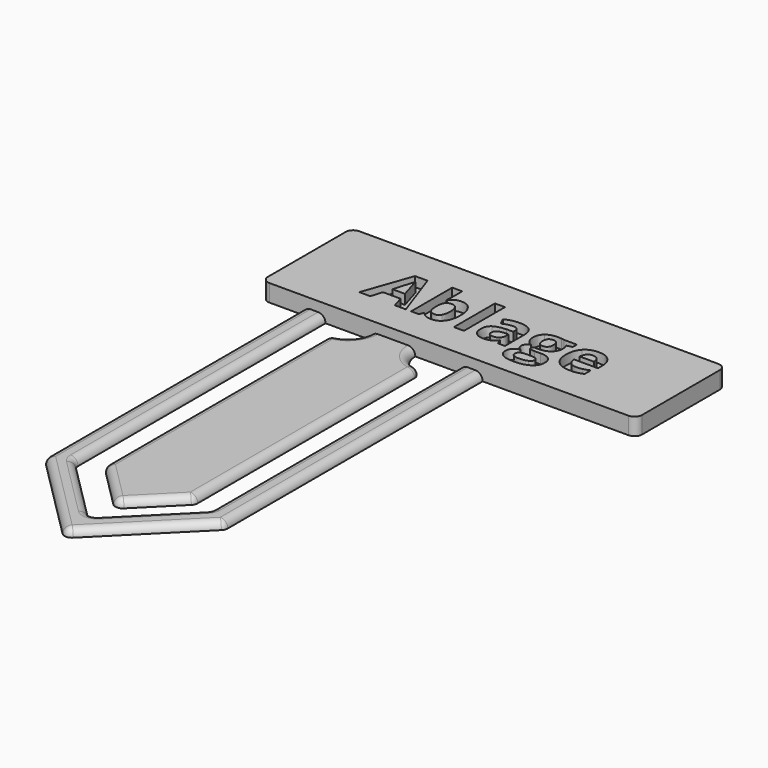
from build123d import *

# Parameters (mm, degrees)
F0_TEXT_SIZE = 9.0277777778
F1_DEPTH     = 1
F0_W         = 1.3442925347
F0_H         = 6.8597005208
F2_DEPTH     = 2.3
F3_R         = 0.99999


# Not quite as in the source:
# - a fillet or chamfer is up to 0.001 mm smaller than in the source, because OpenCascade refuses the exact size
# - Text() gives the source's letters only with a copy of the font that has no kerning and outlines rounded to 1/6400 em; it was checked with that copy


with BuildPart() as f1:
    # F0 (on Top) → F1 (new body)
    with BuildSketch(Plane.XY):
        Polygon((-11.1783012444, 18.0121831276), (-14.1783012444, 18.0121831276), (-14.1783012444, -24.9878168724), (-2.1783012444, -36.9878168724), (9.8216987556, -24.9878168724), (9.8216987556, 18.0121831276), (6.8216987556, 18.0121831276), (6.8216987556, -23.7451761852), (-2.1783012444, -32.7451761852), (-11.1783012444, -23.7451761852), align=None)
        with BuildLine():
            Line((0.8216987556, 18.0121831276), (-5.1783012444, 18.0121831276))
            ThreePointArc((-5.1783012444, 18.0121831276), (-6.0569809009, 15.8908627841), (-8.1783012444, 15.0121831276))
            Line((-8.1783012444, 15.0121831276), (-8.1783012444, -22.5025354981))
            Line((-8.1783012444, -22.5025354981), (-2.1783012444, -28.5025354981))
            Line((-2.1783012444, -28.5025354981), (3.8216987556, -22.5025354981))
            Line((3.8216987556, -22.5025354981), (3.8216987556, 15.0121831276))
            ThreePointArc((3.8216987556, 15.0121831276), (1.700378412, 15.8908627841), (0.8216987556, 18.0121831276))
        make_face()
        with Locations((-10.0730566365, 22.2621831276)):
            Text('Ablage', F0_TEXT_SIZE, font='Open Sans', font_style=FontStyle.BOLD, text_align=(TextAlign.LEFT, TextAlign.BOTTOM))
    extrude(amount=F1_DEPTH)

    # F0 (on Top) → F2 (join)
    with BuildSketch(Plane.XY):
        Polygon((-19.6821061156, 18.0121831276), (-14.1783012444, 18.0121831276), (-11.1783012444, 18.0121831276), (-5.1783012444, 18.0121831276), (0.8216987556, 18.0121831276), (6.8216987556, 18.0121831276), (9.8216987556, 18.0121831276), (30.3178938844, 18.0121831276), (30.3178938844, 33.0121831276), (-19.6821061156, 33.0121831276), align=None)
        Polygon((-3.8438899698, 22.2621831276), (-5.3165462198, 22.2621831276), (-5.7834516017, 23.7969053499), (-8.1334950045, 23.7969053499), (-8.6004003865, 22.2621831276), (-10.0730566365, 22.2621831276), (-7.7977745184, 28.7339713221), (-6.1276356295, 28.7339713221), align=None, mode=Mode.SUBTRACT)
        with BuildLine():
            add(Edge.make_bspline(
                [(-1.7943022962, 26.5517881624), (-1.3217545531, 27.2824739263), (-0.3964073309, 27.2824739263)],
                knots=[0, 0, 0, 1, 1, 1], degree=2))
            add(Edge.make_bspline(
                [(-0.3964073309, 27.2824739263), (0.476748051, 27.2824739263), (0.9704546483, 26.6018641172)],
                knots=[0, 0, 0, 1, 1, 1], degree=2))
            add(Edge.make_bspline(
                [(0.9704546483, 26.6018641172), (1.4641612455, 25.9212543082), (1.4641612455, 24.7349478846)],
                knots=[0, 0, 0, 1, 1, 1], degree=2))
            add(Edge.make_bspline(
                [(1.4641612455, 24.7349478846), (1.4641612455, 23.5147872943), (0.9549381552, 22.8440516172)],
                knots=[0, 0, 0, 1, 1, 1], degree=2))
            add(Edge.make_bspline(
                [(0.9549381552, 22.8440516172), (0.4457150649, 22.1733159401), (-0.4316720878, 22.1733159401)],
                knots=[0, 0, 0, 1, 1, 1], degree=2))
            add(Edge.make_bspline(
                [(-0.4316720878, 22.1733159401), (-1.300595699, 22.1733159401), (-1.7943022962, 22.8038497943)],
                knots=[0, 0, 0, 1, 1, 1], degree=2))
            Line((-1.7943022962, 22.8038497943), (-1.8859906642, 22.8038497943))
            Line((-1.8859906642, 22.8038497943), (-2.1116851087, 22.2621831276))
            Line((-2.1116851087, 22.2621831276), (-3.1385948309, 22.2621831276))
            Line((-3.1385948309, 22.2621831276), (-3.1385948309, 29.1218836485))
            Line((-3.1385948309, 29.1218836485), (-1.7943022962, 29.1218836485))
            Line((-1.7943022962, 29.1218836485), (-1.7943022962, 27.525095454))
            add(Edge.make_bspline(
                [(-1.7943022962, 27.525095454), (-1.7943022962, 27.2218185443), (-1.8464941365, 26.5517881624)],
                knots=[0, 0, 0, 1, 1, 1], degree=2))
            Line((-1.8464941365, 26.5517881624), (-1.7943022962, 26.5517881624))
        make_face(mode=Mode.SUBTRACT)
        with Locations((3.2464420615, 25.6920333881)):
            Rectangle(F0_W, F0_H, mode=Mode.SUBTRACT)
        with BuildLine():
            Line((13.3526161066, 27.1907855582), (15.0721256552, 27.1907855582))
            Line((15.0721256552, 27.1907855582), (15.0721256552, 26.5066492735))
            Line((15.0721256552, 26.5066492735), (14.3005327733, 26.3091666346))
            add(Edge.make_bspline(
                [(14.3005327733, 26.3091666346), (14.5121213149, 25.9776779193), (14.5121213149, 25.5686067388)],
                knots=[0, 0, 0, 1, 1, 1], degree=2))
            add(Edge.make_bspline(
                [(14.5121213149, 25.5686067388), (14.5121213149, 24.7744444124), (13.9584646309, 24.3315190651)],
                knots=[0, 0, 0, 1, 1, 1], degree=2))
            add(Edge.make_bspline(
                [(13.9584646309, 24.3315190651), (13.4048079469, 23.8885937179), (12.4230371135, 23.8885937179)],
                knots=[0, 0, 0, 1, 1, 1], degree=2))
            Line((12.4230371135, 23.8885937179), (12.1804155858, 23.9026996207))
            Line((12.1804155858, 23.9026996207), (11.9815223566, 23.9238584749))
            add(Edge.make_bspline(
                [(11.9815223566, 23.9238584749), (11.7741655858, 23.7658723638), (11.7741655858, 23.5712109054)],
                knots=[0, 0, 0, 1, 1, 1], degree=2))
            add(Edge.make_bspline(
                [(11.7741655858, 23.5712109054), (11.7741655858, 23.2806293082), (12.5147254816, 23.2806293082)],
                knots=[0, 0, 0, 1, 1, 1], degree=2))
            Line((12.5147254816, 23.2806293082), (13.3526161066, 23.2806293082))
            add(Edge.make_bspline(
                [(13.3526161066, 23.2806293082), (14.1637055163, 23.2806293082), (14.5889984851, 22.9322135096)],
                knots=[0, 0, 0, 1, 1, 1], degree=2))
            add(Edge.make_bspline(
                [(14.5889984851, 22.9322135096), (15.0142914538, 22.583797711), (15.0142914538, 21.9095355582)],
                knots=[0, 0, 0, 1, 1, 1], degree=2))
            add(Edge.make_bspline(
                [(15.0142914538, 21.9095355582), (15.0142914538, 21.0448437179), (14.2934798219, 20.5687694992)],
                knots=[0, 0, 0, 1, 1, 1], degree=2))
            add(Edge.make_bspline(
                [(14.2934798219, 20.5687694992), (13.5726681899, 20.0926952804), (12.2241438844, 20.0926952804)],
                knots=[0, 0, 0, 1, 1, 1], degree=2))
            add(Edge.make_bspline(
                [(12.2241438844, 20.0926952804), (11.1930023913, 20.0926952804), (10.6485145441, 20.4523958013)],
                knots=[0, 0, 0, 1, 1, 1], degree=2))
            add(Edge.make_bspline(
                [(10.6485145441, 20.4523958013), (10.1040266969, 20.8120963221), (10.1040266969, 21.4595572596)],
                knots=[0, 0, 0, 1, 1, 1], degree=2))
            add(Edge.make_bspline(
                [(10.1040266969, 21.4595572596), (10.1040266969, 21.9053037874), (10.3819129816, 22.2050542214)],
                knots=[0, 0, 0, 1, 1, 1], degree=2))
            add(Edge.make_bspline(
                [(10.3819129816, 22.2050542214), (10.6597992663, 22.5048046554), (11.1972341622, 22.6331683707)],
                knots=[0, 0, 0, 1, 1, 1], degree=2))
            add(Edge.make_bspline(
                [(11.1972341622, 22.6331683707), (10.9898773913, 22.7206249679), (10.8354177559, 22.9209287874)],
                knots=[0, 0, 0, 1, 1, 1], degree=2))
            add(Edge.make_bspline(
                [(10.8354177559, 22.9209287874), (10.6809581205, 23.1212326068), (10.6809581205, 23.3469270513)],
                knots=[0, 0, 0, 1, 1, 1], degree=2))
            add(Edge.make_bspline(
                [(10.6809581205, 23.3469270513), (10.6809581205, 23.6290451068), (10.8438812976, 23.8159483186)],
                knots=[0, 0, 0, 1, 1, 1], degree=2))
            add(Edge.make_bspline(
                [(10.8438812976, 23.8159483186), (11.0068044747, 24.0028515304), (11.3157237455, 24.1848176763)],
                knots=[0, 0, 0, 1, 1, 1], degree=2))
            add(Edge.make_bspline(
                [(11.3157237455, 24.1848176763), (10.9278114191, 24.351267329), (10.7007063844, 24.721547277)],
                knots=[0, 0, 0, 1, 1, 1], degree=2))
            add(Edge.make_bspline(
                [(10.7007063844, 24.721547277), (10.4736013497, 25.0918272249), (10.4736013497, 25.595407954)],
                knots=[0, 0, 0, 1, 1, 1], degree=2))
            add(Edge.make_bspline(
                [(10.4736013497, 25.595407954), (10.4736013497, 26.4008550026), (10.998340933, 26.8416644645)],
                knots=[0, 0, 0, 1, 1, 1], degree=2))
            add(Edge.make_bspline(
                [(10.998340933, 26.8416644645), (11.5230805163, 27.2824739263), (12.4977983983, 27.2824739263)],
                knots=[0, 0, 0, 1, 1, 1], degree=2))
            add(Edge.make_bspline(
                [(12.4977983983, 27.2824739263), (12.7051551691, 27.2824739263), (12.9893891101, 27.2450932839)],
                knots=[0, 0, 0, 1, 1, 1], degree=2))
            add(Edge.make_bspline(
                [(12.9893891101, 27.2450932839), (13.273623051, 27.2077126415), (13.3526161066, 27.1907855582)],
                knots=[0, 0, 0, 1, 1, 1], degree=2))
        make_face(mode=Mode.SUBTRACT)
        with BuildLine():
            Line((9.3973209677, 22.2621831276), (8.459278433, 22.2621831276))
            Line((8.459278433, 22.2621831276), (8.1983192316, 22.9322135096))
            Line((8.1983192316, 22.9322135096), (8.1630544747, 22.9322135096))
            add(Edge.make_bspline(
                [(8.1630544747, 22.9322135096), (7.824512808, 22.5048046554), (7.4648122872, 22.3390602978)],
                knots=[0, 0, 0, 1, 1, 1], degree=2))
            add(Edge.make_bspline(
                [(7.4648122872, 22.3390602978), (7.1051117663, 22.1733159401), (6.5281803427, 22.1733159401)],
                knots=[0, 0, 0, 1, 1, 1], degree=2))
            add(Edge.make_bspline(
                [(6.5281803427, 22.1733159401), (5.818653433, 22.1733159401), (5.4109928427, 22.5795659401)],
                knots=[0, 0, 0, 1, 1, 1], degree=2))
            add(Edge.make_bspline(
                [(5.4109928427, 22.5795659401), (5.0033322524, 22.9858159401), (5.0033322524, 23.7348393776)],
                knots=[0, 0, 0, 1, 1, 1], degree=2))
            add(Edge.make_bspline(
                [(5.0033322524, 23.7348393776), (5.0033322524, 24.5191275721), (5.5520518705, 24.8915234054)],
                knots=[0, 0, 0, 1, 1, 1], degree=2))
            add(Edge.make_bspline(
                [(5.5520518705, 24.8915234054), (6.1007714885, 25.2639192388), (7.2066742663, 25.3034157665)],
                knots=[0, 0, 0, 1, 1, 1], degree=2))
            Line((7.2066742663, 25.3034157665), (8.0629025649, 25.3302169818))
            Line((8.0629025649, 25.3302169818), (8.0629025649, 25.5460372943))
            add(Edge.make_bspline(
                [(8.0629025649, 25.5460372943), (8.0629025649, 26.2950607318), (7.2955414538, 26.2950607318)],
                knots=[0, 0, 0, 1, 1, 1], degree=2))
            add(Edge.make_bspline(
                [(7.2955414538, 26.2950607318), (6.7045041274, 26.2950607318), (5.9061100302, 25.9381813915)],
                knots=[0, 0, 0, 1, 1, 1], degree=2))
            Line((5.9061100302, 25.9381813915), (5.4617740927, 26.8466015304))
            add(Edge.make_bspline(
                [(5.4617740927, 26.8466015304), (6.3123600302, 27.2923480582), (7.3477332941, 27.2923480582)],
                knots=[0, 0, 0, 1, 1, 1], degree=2))
            add(Edge.make_bspline(
                [(7.3477332941, 27.2923480582), (8.3393782594, 27.2923480582), (8.8683496135, 26.8600021381)],
                knots=[0, 0, 0, 1, 1, 1], degree=2))
            add(Edge.make_bspline(
                [(8.8683496135, 26.8600021381), (9.3973209677, 26.4276562179), (9.3973209677, 25.5460372943)],
                knots=[0, 0, 0, 1, 1, 1], degree=2))
            Line((9.3973209677, 25.5460372943), (9.3973209677, 22.2621831276))
        make_face(mode=Mode.SUBTRACT)
        with BuildLine():
            add(Edge.make_bspline(
                [(19.0923079469, 22.2593619471), (18.691700308, 22.1733159401), (18.1133582941, 22.1733159401)],
                knots=[0, 0, 0, 1, 1, 1], degree=2))
            add(Edge.make_bspline(
                [(18.1133582941, 22.1733159401), (16.9242306899, 22.1733159401), (16.254200308, 22.8306510096)],
                knots=[0, 0, 0, 1, 1, 1], degree=2))
            add(Edge.make_bspline(
                [(16.254200308, 22.8306510096), (15.584169926, 23.487986079), (15.584169926, 24.691219586)],
                knots=[0, 0, 0, 1, 1, 1], degree=2))
            add(Edge.make_bspline(
                [(15.584169926, 24.691219586), (15.584169926, 25.9297178499), (16.203419058, 26.6060958881)],
                knots=[0, 0, 0, 1, 1, 1], degree=2))
            add(Edge.make_bspline(
                [(16.203419058, 26.6060958881), (16.8226681899, 27.2824739263), (17.9158756552, 27.2824739263)],
                knots=[0, 0, 0, 1, 1, 1], degree=2))
            add(Edge.make_bspline(
                [(17.9158756552, 27.2824739263), (18.9597124608, 27.2824739263), (19.5415809503, 26.6879101242)],
                knots=[0, 0, 0, 1, 1, 1], degree=2))
            add(Edge.make_bspline(
                [(19.5415809503, 26.6879101242), (20.1234494399, 26.0933463221), (20.1234494399, 25.0438671554)],
                knots=[0, 0, 0, 1, 1, 1], degree=2))
            Line((20.1234494399, 25.0438671554), (20.1234494399, 24.3907638568))
            Line((20.1234494399, 24.3907638568), (16.9453895441, 24.3907638568))
            add(Edge.make_bspline(
                [(16.9453895441, 24.3907638568), (16.9679589885, 23.818064204), (17.285341801, 23.4964496207)],
                knots=[0, 0, 0, 1, 1, 1], degree=2))
            add(Edge.make_bspline(
                [(17.285341801, 23.4964496207), (17.6027246135, 23.1748350374), (18.1754242663, 23.1748350374)],
                knots=[0, 0, 0, 1, 1, 1], degree=2))
            add(Edge.make_bspline(
                [(18.1754242663, 23.1748350374), (18.6211707941, 23.1748350374), (19.0175466622, 23.2672287006)],
                knots=[0, 0, 0, 1, 1, 1], degree=2))
            add(Edge.make_bspline(
                [(19.0175466622, 23.2672287006), (19.4139225302, 23.3596223638), (19.8455631552, 23.5627473638)],
                knots=[0, 0, 0, 1, 1, 1], degree=2))
            Line((19.8455631552, 23.5627473638), (19.8455631552, 22.5217317388))
            add(Edge.make_bspline(
                [(19.8455631552, 22.5217317388), (19.4929155858, 22.345407954), (19.0923079469, 22.2593619471)],
                knots=[0, 0, 0, 1, 1, 1], degree=2))
        make_face(mode=Mode.SUBTRACT)
        with BuildLine():
            Line((-7.7893109767, 24.9423046554), (-6.1107085462, 24.9423046554))
            add(Edge.make_bspline(
                [(-6.1107085462, 24.9423046554), (-6.7581694837, 27.027157086), (-6.8399837198, 27.3008115999)],
                knots=[0, 0, 0, 1, 1, 1], degree=2))
            add(Edge.make_bspline(
                [(-6.8399837198, 27.3008115999), (-6.9217979559, 27.5744661138), (-6.9570627128, 27.7324522249)],
                knots=[0, 0, 0, 1, 1, 1], degree=2))
            add(Edge.make_bspline(
                [(-6.9570627128, 27.7324522249), (-7.1023535115, 27.1682161138), (-7.7893109767, 24.9423046554)],
                knots=[0, 0, 0, 1, 1, 1], degree=2))
        make_face()
        with BuildLine():
            add(Edge.make_bspline(
                [(-0.1537858031, 25.8436718429), (-0.4006391017, 26.2076041346), (-0.8280479559, 26.2076041346)],
                knots=[0, 0, 0, 1, 1, 1], degree=2))
            add(Edge.make_bspline(
                [(-0.8280479559, 26.2076041346), (-1.3273969142, 26.2076041346), (-1.5566178344, 25.9015060443)],
                knots=[0, 0, 0, 1, 1, 1], degree=2))
            add(Edge.make_bspline(
                [(-1.5566178344, 25.9015060443), (-1.7858387545, 25.595407954), (-1.7943022962, 24.8901128151)],
                knots=[0, 0, 0, 1, 1, 1], degree=2))
            Line((-1.7943022962, 24.8901128151), (-1.7943022962, 24.7434114263))
            add(Edge.make_bspline(
                [(-1.7943022962, 24.7434114263), (-1.7943022962, 23.9506596901), (-1.5580284247, 23.6064756624)],
                knots=[0, 0, 0, 1, 1, 1], degree=2))
            add(Edge.make_bspline(
                [(-1.5580284247, 23.6064756624), (-1.3217545531, 23.2622916346), (-0.8111208726, 23.2622916346)],
                knots=[0, 0, 0, 1, 1, 1], degree=2))
            add(Edge.make_bspline(
                [(-0.8111208726, 23.2622916346), (-0.3964073309, 23.2622916346), (-0.1516699177, 23.6438563047)],
                knots=[0, 0, 0, 1, 1, 1], degree=2))
            add(Edge.make_bspline(
                [(-0.1516699177, 23.6438563047), (0.0930674955, 24.0254209749), (0.0930674955, 24.7532855582)],
                knots=[0, 0, 0, 1, 1, 1], degree=2))
            add(Edge.make_bspline(
                [(0.0930674955, 24.7532855582), (0.0930674955, 25.4797395513), (-0.1537858031, 25.8436718429)],
                knots=[0, 0, 0, 1, 1, 1], degree=2))
        make_face()
        with BuildLine():
            Line((8.0629025649, 24.1396787874), (8.0629025649, 24.5459287874))
            Line((8.0629025649, 24.5459287874), (7.5423947524, 24.5275911138))
            add(Edge.make_bspline(
                [(7.5423947524, 24.5275911138), (6.9555891969, 24.5106640304), (6.6692393705, 24.3167078672)],
                knots=[0, 0, 0, 1, 1, 1], degree=2))
            add(Edge.make_bspline(
                [(6.6692393705, 24.3167078672), (6.3828895441, 24.122751704), (6.3828895441, 23.726375836)],
                knots=[0, 0, 0, 1, 1, 1], degree=2))
            add(Edge.make_bspline(
                [(6.3828895441, 23.726375836), (6.3828895441, 23.1564973638), (7.0345822524, 23.1564973638)],
                knots=[0, 0, 0, 1, 1, 1], degree=2))
            add(Edge.make_bspline(
                [(7.0345822524, 23.1564973638), (7.5028982247, 23.1564973638), (7.7829003948, 23.4259201068)],
                knots=[0, 0, 0, 1, 1, 1], degree=2))
            add(Edge.make_bspline(
                [(7.7829003948, 23.4259201068), (8.0629025649, 23.6953428499), (8.0629025649, 24.1396787874)],
                knots=[0, 0, 0, 1, 1, 1], degree=2))
        make_face()
        with BuildLine():
            add(Edge.make_bspline(
                [(12.4977983983, 26.4671527457), (11.7572385024, 26.4671527457), (11.7572385024, 25.5770702804)],
                knots=[0, 0, 0, 1, 1, 1], degree=2))
            add(Edge.make_bspline(
                [(11.7572385024, 25.5770702804), (11.7572385024, 25.1764626415), (11.9399099434, 24.9423046554)],
                knots=[0, 0, 0, 1, 1, 1], degree=2))
            add(Edge.make_bspline(
                [(11.9399099434, 24.9423046554), (12.1225813844, 24.7081466693), (12.4977983983, 24.7081466693)],
                knots=[0, 0, 0, 1, 1, 1], degree=2))
            add(Edge.make_bspline(
                [(12.4977983983, 24.7081466693), (12.8758365927, 24.7081466693), (13.0521603774, 24.9423046554)],
                knots=[0, 0, 0, 1, 1, 1], degree=2))
            add(Edge.make_bspline(
                [(13.0521603774, 24.9423046554), (13.2284841622, 25.1764626415), (13.2284841622, 25.5770702804)],
                knots=[0, 0, 0, 1, 1, 1], degree=2))
            add(Edge.make_bspline(
                [(13.2284841622, 25.5770702804), (13.2284841622, 26.4671527457), (12.4977983983, 26.4671527457)],
                knots=[0, 0, 0, 1, 1, 1], degree=2))
        make_face()
        with BuildLine():
            add(Edge.make_bspline(
                [(11.5167328601, 22.0259092561), (11.267763676, 21.8517013568), (11.267763676, 21.5653515304)],
                knots=[0, 0, 0, 1, 1, 1], degree=2))
            add(Edge.make_bspline(
                [(11.267763676, 21.5653515304), (11.267763676, 21.2874652457), (11.5343652385, 21.1287738395)],
                knots=[0, 0, 0, 1, 1, 1], degree=2))
            add(Edge.make_bspline(
                [(11.5343652385, 21.1287738395), (11.800966801, 20.9700824332), (12.2819780858, 20.9700824332)],
                knots=[0, 0, 0, 1, 1, 1], degree=2))
            add(Edge.make_bspline(
                [(12.2819780858, 20.9700824332), (13.004200308, 20.9700824332), (13.4139767837, 21.1689756624)],
                knots=[0, 0, 0, 1, 1, 1], degree=2))
            add(Edge.make_bspline(
                [(13.4139767837, 21.1689756624), (13.8237532594, 21.3678688915), (13.8237532594, 21.710642329)],
                knots=[0, 0, 0, 1, 1, 1], degree=2))
            add(Edge.make_bspline(
                [(13.8237532594, 21.710642329), (13.8237532594, 21.9885286138), (13.5818370267, 22.0943228846)],
                knots=[0, 0, 0, 1, 1, 1], degree=2))
            add(Edge.make_bspline(
                [(13.5818370267, 22.0943228846), (13.3399207941, 22.2001171554), (12.8321082941, 22.2001171554)],
                knots=[0, 0, 0, 1, 1, 1], degree=2))
            Line((12.8321082941, 22.2001171554), (12.1352766969, 22.2001171554))
            add(Edge.make_bspline(
                [(12.1352766969, 22.2001171554), (11.7657020441, 22.2001171554), (11.5167328601, 22.0259092561)],
                knots=[0, 0, 0, 1, 1, 1], degree=2))
        make_face()
        with BuildLine():
            add(Edge.make_bspline(
                [(18.6028331205, 26.0552603846), (18.351748051, 26.3260937179), (17.9243391969, 26.3260937179)],
                knots=[0, 0, 0, 1, 1, 1], degree=2))
            add(Edge.make_bspline(
                [(17.9243391969, 26.3260937179), (17.4969303427, 26.3260937179), (17.2543088149, 26.0552603846)],
                knots=[0, 0, 0, 1, 1, 1], degree=2))
            add(Edge.make_bspline(
                [(17.2543088149, 26.0552603846), (17.0116872872, 25.7844270513), (16.9764225302, 25.2864886832)],
                knots=[0, 0, 0, 1, 1, 1], degree=2))
            Line((16.9764225302, 25.2864886832), (18.8637923219, 25.2864886832))
            add(Edge.make_bspline(
                [(18.8637923219, 25.2864886832), (18.8539181899, 25.7844270513), (18.6028331205, 26.0552603846)],
                knots=[0, 0, 0, 1, 1, 1], degree=2))
        make_face()
    extrude(amount=F2_DEPTH)

    # F3 (radius 1 in the source; OpenCascade refuses exactly that, so slightly less here)
    f3_edges = [f1.edges().sort_by_distance(p)[0] for p in [
        (-19.682106, 33.012183, 1.15),
        (-19.682106, 18.012183, 1.15),
        (-8.178301, 15.012183, 0.5),
        (-8.178301, -22.502535, 0.5),
        (-14.178301, -24.987817, 0.5),
        (-2.178301, -28.502535, 0.5),
        (-2.178301, -36.987817, 0.5),
        (6.821699, -23.745176, 0.5),
        (3.821699, 15.012183, 0.5),
        (30.317894, 18.012183, 1.15),
        (30.317894, 33.012183, 1.15),
        (9.821699, -24.987817, 0.5),
        (3.821699, -22.502535, 0.5),
        (-11.178301, -23.745176, 0.5),
        (-2.178301, -32.745176, 0.5),
        (3.821699, -30.987817, 1),
        (9.821699, -3.487817, 1),
        (-8.178301, -30.987817, 1),
        (-14.178301, -3.487817, 1),
        (-5.178301, -25.502535, 1),
        (0.821699, -25.502535, 1),
        (3.821699, -3.745176, 1),
        (-8.178301, -3.745176, 1),
        (-11.178301, -2.866497, 1),
        (1.700378, 15.890863, 1),
        (-6.056981, 15.890863, 1),
        (6.821699, -2.866497, 1),
        (2.321699, -28.245176, 1),
        (-6.678301, -28.245176, 1),
    ]]
    fillet(f3_edges, radius=F3_R)


solid = f1.part
